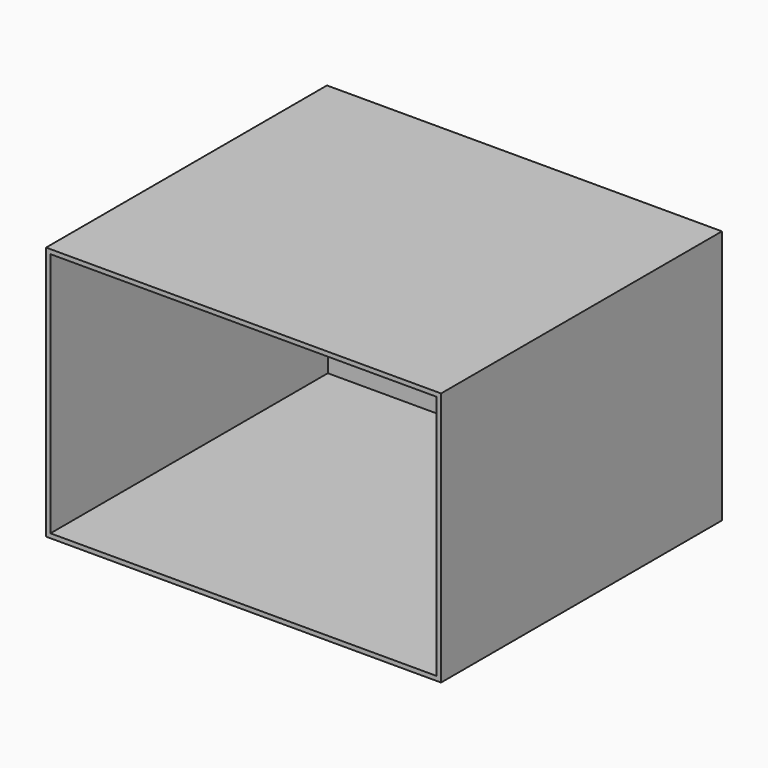
from build123d import *

# Parameters (mm, degrees)
F0_W     = 571.5
F0_H     = 368.3
F0_W_2   = 558.8
F0_H_2   = 355.6
F1_DEPTH = 508
F2_START = -501.65
F2_DEPTH = 6.35


with BuildPart() as f1:
    # F0 (on Front) → F1 (new body)
    with BuildSketch(Plane.XZ):
        Rectangle(F0_W, F0_H)
        Rectangle(F0_W_2, F0_H_2, mode=Mode.SUBTRACT)
    extrude(amount=-F1_DEPTH)


with BuildPart() as f2:
    # F0 (on Front) → F2 (new body)
    with BuildSketch(Plane.XZ.offset(F2_START)):
        Rectangle(F0_W_2, F0_H_2)
    extrude(amount=-F2_DEPTH)


solid = Compound([f1.part, f2.part])
